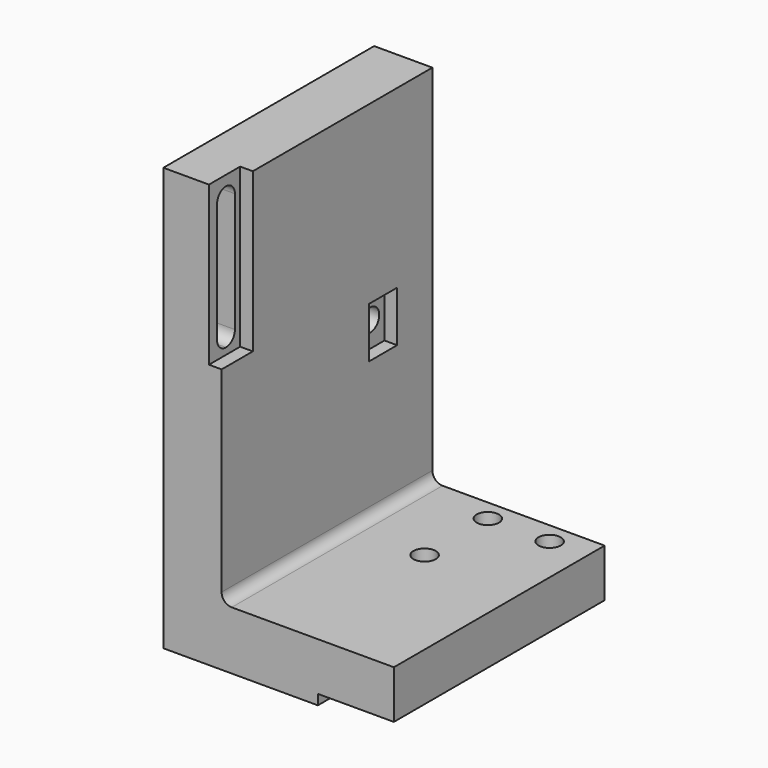
from build123d import *

# Parameters (mm, degrees)
F0_W        = 45.5
F0_H        = 83.5
F1_DEPTH    = 52
F2_W        = 34
F2_H        = 72
F3_DEPTH    = 52.001
F5_W        = 15
F5_H        = 2
F6_DEPTH    = 52.001
F8_R        = 2
F10_D       = 4.4
F10_ON_F9_D = 4.4
F10_ON_F4_D = 4.4
F12_DEPTH   = 45.501
F13_W       = 7
F13_H       = 10
F14_DEPTH   = 2.5
F15_W       = 7.7
F15_H       = 31.3
F16_DEPTH   = 2.5


# Not quite as in the source:
# - a feature names something its author has since deleted; it is built from what else it names


with BuildPart() as f1:
    # F0 (on Front) → F1 (new body)
    with BuildSketch(Plane.XZ):
        with Locations((11.25, 30.25)):
            Rectangle(F0_W, F0_H)
    extrude(amount=F1_DEPTH)

    # F2 (on face) → F3 (cut, through all)
    with BuildSketch(Plane.XZ.offset(52)):
        with Locations((17, 36)):
            Rectangle(F2_W, F2_H)
    extrude(amount=-F3_DEPTH, mode=Mode.SUBTRACT)

    # F5 (on face) → F6 (cut, through all)
    with BuildSketch(Plane.XZ.offset(52)):
        with Locations((26.5, -10.5)):
            Rectangle(F5_W, F5_H)
    extrude(amount=-F6_DEPTH, mode=Mode.SUBTRACT)

    # F8
    f8_edges = [f1.edges().sort_by_distance(p)[0] for p in [
        (0, -26, 0),
    ]]
    fillet(f8_edges, radius=F8_R)

    # F10 (through all)
    with Locations(Plane.XY):
        with Locations((26.5, -4.2)):
            Hole(F10_D / 2)

    # F10 on F9 (through all)
    with Locations(Plane(origin=(-11.5, 0, 0), x_dir=(0, -1, 0), z_dir=(-1, 0, 0))):
        with Locations((12.2, 32.3)):
            Hole(F10_ON_F9_D / 2)

    # F10 on F4 (through all)
    with Locations(Plane(origin=(0, 0, -11.5), x_dir=(1, 0, 0), z_dir=(0, 0, -1))):
        with Locations((14.3, 19.8), (14.3, 4.2)):
            Hole(F10_ON_F4_D / 2)

    # F11 (on face) → F12 (cut, through all)
    with BuildSketch(Plane(origin=(-11.5, 0, 0), x_dir=(0, -1, 0), z_dir=(-1, 0, 0))):
        with BuildLine():
            ThreePointArc((47.8, 70), (46.2443650814, 69.3556349186), (45.6, 67.8))
            Line((45.6, 67.8), (45.6, 44.2))
            ThreePointArc((45.6, 44.2), (46.2443650814, 42.6443650814), (47.8, 42))
            ThreePointArc((47.8, 42), (49.3556349186, 42.6443650814), (50, 44.2))
            Line((50, 44.2), (50, 67.8))
            ThreePointArc((50, 67.8), (49.3556349186, 69.3556349186), (47.8, 70))
        make_face()
    extrude(amount=-F12_DEPTH, mode=Mode.SUBTRACT)

    # F13 (on face) → F14 (cut)
    with BuildSketch(Plane.YZ):
        with Locations((-12.2, 32.3)):
            Rectangle(F13_W, F13_H)
    extrude(amount=-F14_DEPTH, mode=Mode.SUBTRACT)

    # F15 (on face) → F16 (cut)
    with BuildSketch(Plane.YZ):
        with Locations((-48.15, 56.35)):
            Rectangle(F15_W, F15_H)
        with BuildLine():
            Line((-50, 44.2), (-50, 67.8))
            ThreePointArc((-50, 67.8), (-47.8, 70), (-45.6, 67.8))
            Line((-45.6, 67.8), (-45.6, 44.2))
            ThreePointArc((-45.6, 44.2), (-47.8, 42), (-50, 44.2))
        make_face(mode=Mode.SUBTRACT)
    extrude(amount=-F16_DEPTH, mode=Mode.SUBTRACT)


solid = f1.part
